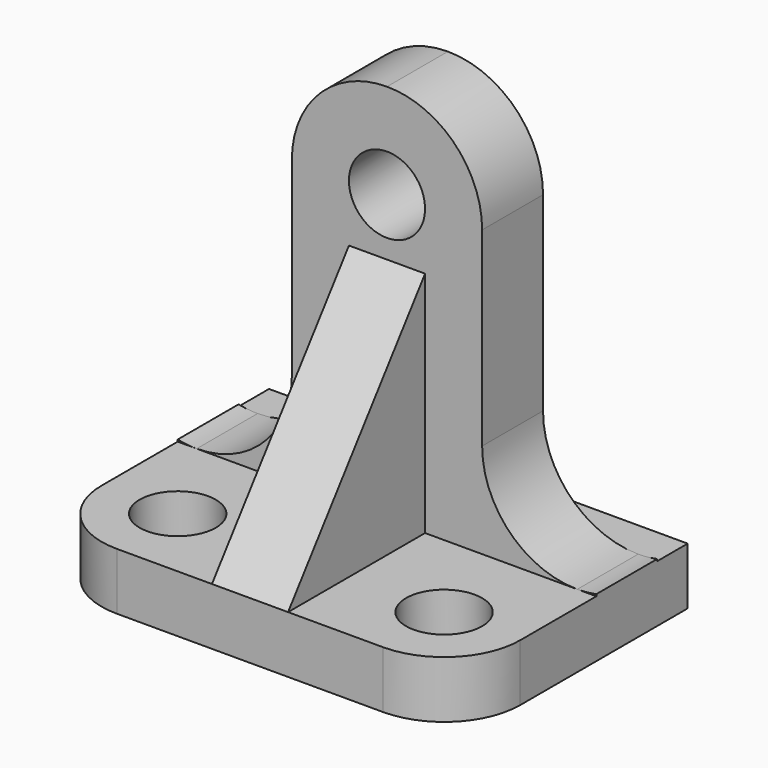
from build123d import *

# Parameters (mm, degrees)
F0_W         = 110
F0_H         = 75
F1_DEPTH     = 115
F2_W         = 10
F2_H         = 100
F3_DEPTH     = 110.001
F4_R         = 10
F5_DEPTH     = 65.001
F6_R         = 10
F7_DEPTH     = 115.001
F9_DEPTH     = 45
F11_DEPTH    = 65.001
F12_T1_DEPTH = 115.5051025722
F12_T3_DEPTH = 115
F14_DEPTH    = 45.0010001
F16_DEPTH    = 45.0010001


# Not quite as in the source:
# - a fillet or chamfer that OpenCascade refuses, or shapes differently, is made with other operations: its cross-section is extruded or revolved along the edge and cut away or added


with BuildPart() as f1:
    # F0 (on Top) → F1 (new body)
    with BuildSketch(Plane.XY):
        with Locations((55, -37.5)):
            Rectangle(F0_W, F0_H)
    extrude(amount=F1_DEPTH)

    # F2 (on face) → F3 (cut, through all)
    with BuildSketch(Plane.YZ.offset(110)):
        with Locations((-5, 65)):
            Rectangle(F2_W, F2_H)
    extrude(amount=-F3_DEPTH, mode=Mode.SUBTRACT)

    # F4 (on face) → F5 (cut, through all)
    with BuildSketch(Plane(origin=(0, -10, 0), x_dir=(-1, 0, 0), z_dir=(0, 1, 0))):
        with BuildLine():
            ThreePointArc((-110, 64.4948974278), (-89.1886116992, 59.364916731), (-80, 40))
            Line((-80, 40), (-80, 90))
            Line((-80, 90), (-80, 115))
            Line((-80, 115), (-110, 115))
            Line((-110, 115), (-110, 64.4948974278))
        make_face()
        with BuildLine():
            ThreePointArc((-105, 15), (-87.3223304703, 22.3223304703), (-80, 40))
            ThreePointArc((-80, 40), (-89.1886116992, 59.364916731), (-110, 64.4948974278))
            Line((-110, 64.4948974278), (-110, 15.5051025722))
            ThreePointArc((-110, 15.5051025722), (-107.5127240501, 15.1265961749), (-105, 15))
        make_face()
        with BuildLine():
            ThreePointArc((0, 64.4948974278), (-20.8113883008, 59.364916731), (-30, 40))
            ThreePointArc((-30, 40), (-22.6776695035, 22.3223304441), (-4.9999999259, 15))
            ThreePointArc((-4.9999999259, 15), (-2.487275913, 15.1265961786), (0, 15.5051025722))
            Line((0, 15.5051025722), (0, 64.4948974278))
        make_face()
        with BuildLine():
            Line((-30, 90), (-30, 40))
            ThreePointArc((-30, 40), (-20.8113883008, 59.364916731), (0, 64.4948974278))
            Line((0, 64.4948974278), (0, 115))
            Line((0, 115), (-30, 115))
            Line((-30, 115), (-30, 90))
        make_face()
        with BuildLine():
            ThreePointArc((-55, 115), (-37.3223304703, 107.6776695297), (-30, 90))
            Line((-30, 90), (-30, 115))
            Line((-30, 115), (-55, 115))
        make_face()
        with BuildLine():
            Line((-80, 115), (-80, 90))
            ThreePointArc((-80, 90), (-72.6776695297, 107.6776695297), (-55, 115))
            Line((-55, 115), (-80, 115))
        make_face()
        with Locations((-55, 90)):
            Circle(F4_R)
    extrude(amount=-F5_DEPTH, mode=Mode.SUBTRACT)

    # F6 (on face) → F7 (cut, through all)
    with BuildSketch(Plane(origin=(0, 0, 0), x_dir=(1, 0, 0), z_dir=(0, 0, -1))):
        with Locations((90, 55)):
            Circle(F6_R)
        with Locations((20, 55)):
            Circle(F6_R)
    extrude(amount=-F7_DEPTH, mode=Mode.SUBTRACT)

    # F8 (on face) → F9 (cut)
    with BuildSketch(Plane.XZ.offset(75)):
        with BuildLine():
            Line((0, 115), (0, 15.5051025722))
            ThreePointArc((0, 15.5051025722), (2.4872759548, 15.1265961744), (5.00000001, 15))
            ThreePointArc((5.00000001, 15), (22.6776695332, 22.3223304739), (30, 40))
            Line((30, 40), (30, 90))
            ThreePointArc((30, 90), (34.0834993366, 103.6930639376), (45, 112.9128784748))
            Line((45, 112.9128784748), (45, 115))
            Line((45, 115), (0, 115))
        make_face()
        with BuildLine():
            ThreePointArc((30, 40), (22.6776695332, 22.3223304739), (5.00000001, 15))
            Line((5.00000001, 15), (45, 15))
            Line((45, 15), (45, 75))
            Line((45, 75), (45, 90))
            Line((45, 90), (45, 112.9128784748))
            ThreePointArc((45, 112.9128784748), (34.0834993366, 103.6930639376), (30, 90))
            Line((30, 90), (30, 40))
        make_face()
        with BuildLine():
            ThreePointArc((105.0000000223, 15), (107.5127240612, 15.126596176), (110, 15.5051025722))
            Line((110, 15.5051025722), (110, 115))
            Line((110, 115), (65, 115))
            Line((65, 115), (65, 112.9128784748))
            ThreePointArc((65, 112.9128784748), (75.9165006634, 103.6930639376), (80, 90))
            Line((80, 90), (80, 40))
            ThreePointArc((80, 40), (87.3223304782, 22.3223304625), (105.0000000223, 15))
        make_face()
        with BuildLine():
            Line((65, 15), (105.0000000223, 15))
            ThreePointArc((105.0000000223, 15), (87.3223304782, 22.3223304625), (80, 40))
            Line((80, 40), (80, 90))
            ThreePointArc((80, 90), (75.9165006634, 103.6930639376), (65, 112.9128784748))
            Line((65, 112.9128784748), (65, 90))
            Line((65, 90), (65, 75))
            Line((65, 75), (65, 15))
        make_face()
        with BuildLine():
            Line((45, 90), (45, 75))
            Line((45, 75), (65, 75))
            Line((65, 75), (65, 90))
            ThreePointArc((65, 90), (55, 80), (45, 90))
        make_face()
        with BuildLine():
            ThreePointArc((65, 112.9128784748), (60.1077410922, 114.4726578233), (55, 115))
            ThreePointArc((55, 115), (49.8922589078, 114.4726578233), (45, 112.9128784748))
            Line((45, 112.9128784748), (45, 90))
            ThreePointArc((45, 90), (55, 100), (65, 90))
            Line((65, 90), (65, 112.9128784748))
        make_face()
        with BuildLine():
            ThreePointArc((65, 90), (55, 100), (45, 90))
            ThreePointArc((45, 90), (55, 80), (65, 90))
        make_face()
    extrude(amount=-F9_DEPTH, mode=Mode.SUBTRACT)

    # F10 (on face) → F11 (cut, through all)
    with BuildSketch(Plane.YZ.offset(65)):
        Polygon((-75, 75), (-75, 15), (-30, 75), align=None)
    extrude(amount=-F11_DEPTH, mode=Mode.SUBTRACT)

    # F12: fillet of radius 20 on 2 edges, made by hand

    # F12_s2 → F12_t1 (cut)
    with BuildSketch(Plane.XY.offset(-50)):
        with BuildLine():
            ThreePointArc((110, -55), (104.1421356237, -69.1421356237), (90, -75))
            Line((90, -75), (110, -75))
            Line((110, -75), (110, -55))
        make_face()
    extrude(amount=F12_T1_DEPTH, mode=Mode.SUBTRACT)

    # F12_s4 → F12_t3 (cut)
    with BuildSketch(Plane.XY.offset(-50)):
        with BuildLine():
            ThreePointArc((20, -75), (5.8578643763, -69.1421356237), (0, -55))
            Line((0, -55), (0, -75))
            Line((0, -75), (20, -75))
        make_face()
    extrude(amount=F12_T3_DEPTH, mode=Mode.SUBTRACT)

    # F14 (cut, through all): a face of the model
    f14_faces = [f1.faces().sort_by_distance(p)[0] for p in [
        (65, -45, 35),
    ]]
    extrude(f14_faces, amount=F14_DEPTH, mode=Mode.SUBTRACT)

    # F15 (on face) → F16 (cut, through all)
    with BuildSketch(Plane(origin=(45, 0, 0), x_dir=(0, -1, 0), z_dir=(-1, 0, 0))):
        Polygon((30, 75), (30, 15), (75, 15), align=None)
    extrude(amount=F16_DEPTH, mode=Mode.SUBTRACT)


solid = f1.part
